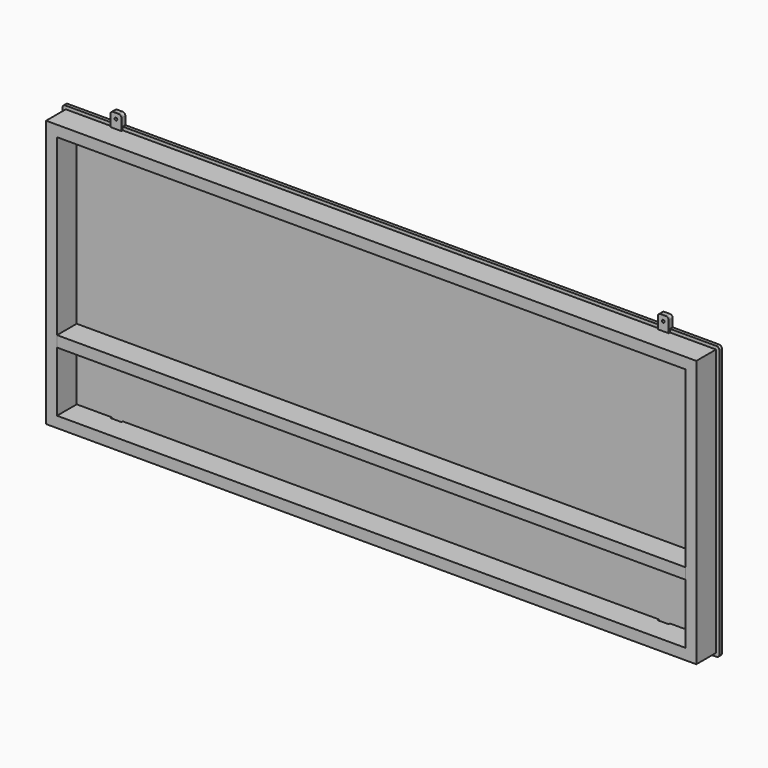
from build123d import *

# Parameters (mm, degrees)
F0_W      = 20
F0_H      = 448
F1_DEPTH  = 45
F2_W      = 20
F2_H      = 20
F2_R      = 2.5
F3_DEPTH  = 6
F4_W      = 1148
F4_H      = 20
F5_DEPTH  = 45
F6_R      = 5
F7_R      = 5
F8_W      = 20
F8_H      = 3
F9_DEPTH  = 25
F10_W     = 20
F10_H     = 40
F10_R     = 2.5
F11_DEPTH = 3
F12_R     = 5
F13_W     = 20
F13_H     = 3
F14_DEPTH = 25
F15_R     = 5
F15_2_R   = 5
F16_R     = 5


with BuildPart() as f1:
    # F0 (on Front) → F1 (new body)
    with BuildSketch(Plane.XZ):
        Polygon((-594, 223.0578817198), (-594, 203.0578817198), (-574, 203.0578817198), (574, 203.0578817198), (594, 203.0578817198), (594, 223.0578817198), align=None)
        with Locations((-584, -20.9421182802)):
            Rectangle(F0_W, F0_H)
        Polygon((-574, -244.9421182802), (-594, -244.9421182802), (-594, -264.9421182802), (594, -264.9421182802), (594, -244.9421182802), (574, -244.9421182802), align=None)
        with Locations((584, -20.9421182802)):
            Rectangle(F0_W, F0_H)
    extrude(amount=F1_DEPTH)

    # F8 (on face) → F9 (cut)
    with BuildSketch(Plane.XY.offset(223.0578817198)):
        with Locations((-500.0000202656, -1.5)):
            Rectangle(F8_W, F8_H)
        with Locations((500.0000202656, -1.5)):
            Rectangle(F8_W, F8_H)
    extrude(amount=-F9_DEPTH, mode=Mode.SUBTRACT)


with BuildPart() as f3:
    # F2 (on face) → F3 (new body)
    with BuildSketch(Plane(origin=(0, 0, 0), x_dir=(-1, 0, 0), z_dir=(0, 1, 0))):
        Polygon((-510, 229.0578817198), (-600, 229.0578817198), (-600, -270.9421182802), (-510, -270.9421182802), (-510, -250.9421182802), (-490, -250.9421182802), (-490, -270.9421182802), (490, -270.9421182802), (490, -250.9421182802), (510, -250.9421182802), (510, -270.9421182802), (600, -270.9421182802), (600, 229.0578817198), (510, 229.0578817198), (510, 209.0578817198), (490, 209.0578817198), (490, 229.0578817198), (-490, 229.0578817198), (-490, 209.0578817198), (-510, 209.0578817198), align=None)
        with Locations((-500, 239.0578817198)):
            Rectangle(F2_W, F2_H)
        with Locations((-500, 239.0578817198)):
            Circle(F2_R, mode=Mode.SUBTRACT)
        with Locations((-500, 219.0578817198)):
            Rectangle(F2_W, F2_H)
        with Locations((-500, 219.0578817198)):
            Circle(F2_R, mode=Mode.SUBTRACT)
        with Locations((-500, -260.9421182802)):
            Rectangle(F2_W, F2_H)
        with Locations((-500, -260.9421182802)):
            Circle(F2_R, mode=Mode.SUBTRACT)
        with Locations((-500, -280.9421182802)):
            Rectangle(F2_W, F2_H)
        with Locations((-500, -280.9421182802)):
            Circle(F2_R, mode=Mode.SUBTRACT)
        with Locations((500, 239.0578817198)):
            Rectangle(F2_W, F2_H)
        with Locations((500, 239.0578817198)):
            Circle(F2_R, mode=Mode.SUBTRACT)
        with Locations((500, 219.0578817198)):
            Rectangle(F2_W, F2_H)
        with Locations((500, 219.0578817198)):
            Circle(F2_R, mode=Mode.SUBTRACT)
        with Locations((500, -260.9421182802)):
            Rectangle(F2_W, F2_H)
        with Locations((500, -260.9421182802)):
            Circle(F2_R, mode=Mode.SUBTRACT)
        with Locations((500, -280.9421182802)):
            Rectangle(F2_W, F2_H)
        with Locations((500, -280.9421182802)):
            Circle(F2_R, mode=Mode.SUBTRACT)
    extrude(amount=F3_DEPTH)

    # F6
    f6_edges = [f3.edges().sort_by_distance(p)[0] for p in [
        (510, 3, 249.057882),
        (490, 3, 249.057882),
    ]]
    fillet(f6_edges, radius=F6_R)

    # F7
    f7_edges = [f3.edges().sort_by_distance(p)[0] for p in [
        (510, 3, -290.942118),
        (490, 3, -290.942118),
        (-510, 3, 249.057882),
        (-490, 3, 249.057882),
        (-510, 3, -290.942118),
        (-490, 3, -290.942118),
        (600, 3, 229.057882),
        (-600, 3, 229.057882),
        (600, 3, -270.942118),
        (-600, 3, -270.942118),
    ]]
    fillet(f7_edges, radius=F7_R)


with BuildPart() as f5:
    # F4 (on face) → F5 (new body)
    with BuildSketch(Plane.XZ):
        with Locations((0, -125.320276022)):
            Rectangle(F4_W, F4_H)
    extrude(amount=F5_DEPTH)


with BuildPart() as f11:
    # F10 (on face) → F11 (new body)
    with BuildSketch(Plane.XZ):
        with Locations((-500, 229.0578817198)):
            Rectangle(F10_W, F10_H)
        with Locations((-500, 219.0578817198)):
            Circle(F10_R, mode=Mode.SUBTRACT)
        with Locations((-500, 239.0578817198)):
            Circle(F10_R, mode=Mode.SUBTRACT)
    extrude(amount=F11_DEPTH)

    # F12
    f12_edges = [f11.edges().sort_by_distance(p)[0] for p in [
        (-510, -1.5, 249.057882),
        (-490, -1.5, 249.057882),
        (-490, -1.5, 209.057882),
        (-510, -1.5, 209.057882),
    ]]
    fillet(f12_edges, radius=F12_R)


with BuildPart() as f11b:
    # F10 (on face) → F11, piece 2 (new body)
    with BuildSketch(Plane.XZ):
        with Locations((500, 229.0578817198)):
            Rectangle(F10_W, F10_H)
        with Locations((500, 219.0578817198)):
            Circle(F10_R, mode=Mode.SUBTRACT)
        with Locations((500, 239.0578817198)):
            Circle(F10_R, mode=Mode.SUBTRACT)
    extrude(amount=F11_DEPTH)

    # F15
    f15_edges = [f11b.edges().sort_by_distance(p)[0] for p in [
        (510, -1.5, 249.057882),
        (490, -1.5, 249.057882),
    ]]
    fillet(f15_edges, radius=F15_R)


with BuildPart() as f11c:
    # F10 (on face) → F11, piece 3 (new body)
    with BuildSketch(Plane.XZ):
        with Locations((-500, -270.9421182802)):
            Rectangle(F10_W, F10_H)
        with Locations((-500, -280.9421182802)):
            Circle(F10_R, mode=Mode.SUBTRACT)
        with Locations((-500, -260.9421182802)):
            Circle(F10_R, mode=Mode.SUBTRACT)
    extrude(amount=F11_DEPTH)


with BuildPart() as f11d:
    # F10 (on face) → F11, piece 4 (new body)
    with BuildSketch(Plane.XZ):
        with Locations((500, -270.9421182802)):
            Rectangle(F10_W, F10_H)
        with Locations((500, -280.9421182802)):
            Circle(F10_R, mode=Mode.SUBTRACT)
        with Locations((500, -260.9421182802)):
            Circle(F10_R, mode=Mode.SUBTRACT)
    extrude(amount=F11_DEPTH)


with BuildPart() as f14_tool:
    # F13 (on face) → F14 (new body)
    with BuildSketch(Plane(origin=(0, 0, -264.9421182802), x_dir=(1, 0, 0), z_dir=(0, 0, -1))):
        with Locations((500, 1.5)):
            Rectangle(F13_W, F13_H)
        with Locations((-500, 1.5)):
            Rectangle(F13_W, F13_H)
    extrude(amount=-F14_DEPTH)


with BuildPart() as f1_1:
    add(f1.part)

    # F14: cut by f14_tool
    add(f14_tool.part, mode=Mode.SUBTRACT)


with BuildPart() as f11c_1:
    add(f11c.part)

    # F14: cut by f14_tool
    add(f14_tool.part, mode=Mode.SUBTRACT)

    # F15#2
    f15_2_edges = [f11c_1.edges().sort_by_distance(p)[0] for p in [
        (-510, -1.5, -290.942118),
        (-490, -1.5, -290.942118),
    ]]
    fillet(f15_2_edges, radius=F15_2_R)


with BuildPart() as f11d_1:
    add(f11d.part)

    # F14: cut by f14_tool
    add(f14_tool.part, mode=Mode.SUBTRACT)

    # F16
    f16_edges = [f11d_1.edges().sort_by_distance(p)[0] for p in [
        (510, -1.5, -290.942118),
        (490, -1.5, -290.942118),
    ]]
    fillet(f16_edges, radius=F16_R)


solid = Compound([f3.part, f5.part, f11.part, f11b.part, f1_1.part, f11c_1.part, f11d_1.part])
